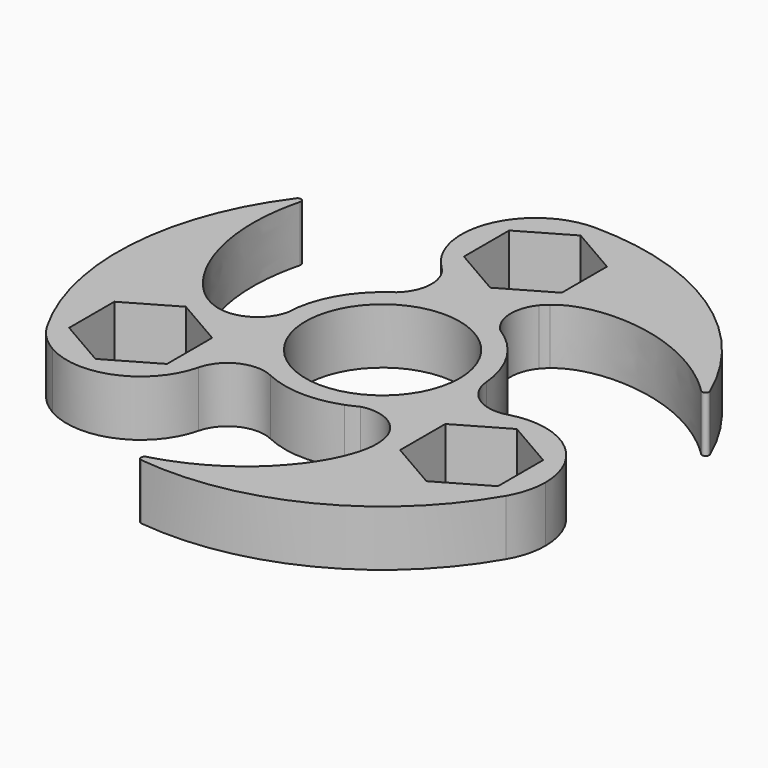
from build123d import *

# Parameters (mm, degrees)
F0_R     = 11.05
F1_DEPTH = 8
F3_R     = 0.5
F4_COUNT = 3


with BuildPart() as f1:
    # F0 (on Top) → F1 (new body)
    with BuildSketch(Plane.XY):
        with BuildLine():
            ThreePointArc((34.3290960637, -13.7), (30.0916651535, -5.2219274255), (20.7672631245, -3.5222033013))
            ThreePointArc((20.7672631245, -3.5222033013), (14.6823659307, -8.1758101137), (13.3222862083, -15.7145244187))
            ThreePointArc((13.3222862083, -15.7145244187), (13.5070330584, -16.3019267518), (13.6256086025, -16.9061723475))
            ThreePointArc((13.6256086025, -16.9061723475), (22.5848514527, -24.2380597963), (32.9089655486, -18.9999996453))
            ThreePointArc((32.9089655486, -18.9999996453), (33.9679098754, -16.4434816803), (34.3290960637, -13.7))
        make_face()
        Polygon((16.714290293, -17.75), (16.714290293, -9.65), (23.7290960637, -5.6), (30.7439018343, -9.65), (30.7439018343, -17.75), (23.7290960637, -21.8), align=None, mode=Mode.SUBTRACT)
        with BuildLine():
            ThreePointArc((32.9089655486, -18.9999996453), (22.5848514527, -24.2380597963), (13.6256086025, -16.9061723475))
            add(Edge.make_bspline(
                [(13.6256086025, -16.9061723475), (14.801474957, -22.8848015035), (7.2970846668, -34.7264185548), (-7.0017315099, -37.3493742366)],
                knots=[0, 0, 0, 0, 29.0415506403, 29.0415506403, 29.0415506403, 29.0415506403], degree=3))
            ThreePointArc((-7.0017315099, -37.3493742366), (15.8735969728, -34.525771811), (32.9089655486, -18.9999996453))
        make_face()
        with BuildLine():
            ThreePointArc((13.9516175859, 1.162913039), (13.9878991668, 0.5819595334), (14, 0))
            ThreePointArc((14, 0), (12.0245892037, -7.1700247198), (6.6558207882, -12.3166574052))
            ThreePointArc((6.6558207882, -12.3166574052), (10.6472554887, -12.7242275975), (13.3222862083, -15.7145244187))
            ThreePointArc((13.3222862083, -15.7145244187), (14.6823659307, -8.1758101137), (20.7672631245, -3.5222033013))
            ThreePointArc((20.7672631245, -3.5222033013), (16.2488562156, -2.7952608995), (13.9516175859, 1.162913039))
        make_face()
        with BuildLine():
            ThreePointArc((6.6558207882, -12.3166574052), (12.0245892037, -7.1700247198), (14, 0))
            ThreePointArc((14, 0), (13.9878991668, 0.5819595334), (13.9516175859, 1.162913039))
            ThreePointArc((13.9516175859, 1.162913039), (-11.8574125056, 7.443236438), (5.0171266013, -13.0701354494))
            ThreePointArc((5.0171266013, -13.0701354494), (5.8056785292, -12.6264218696), (6.6558207882, -12.3166574052))
        make_face()
        Circle(F0_R, mode=Mode.SUBTRACT)
    extrude(amount=F1_DEPTH)

    # F3
    f3_edges = [f1.edges().sort_by_distance(p)[0] for p in [
        (-7.001732, -37.349374, 4),
    ]]
    fillet(f3_edges, radius=F3_R)

    # F4: F1 ×3 about axis
    f4_axis = Axis((0, 0, 2.8210394084), (0, 0, -1))


with BuildPart() as f1_1:
    add(f1.part)
    for i in range(1, F4_COUNT):
        add(f1.part.rotate(f4_axis, i * 360 / F4_COUNT))


solid = f1_1.part
